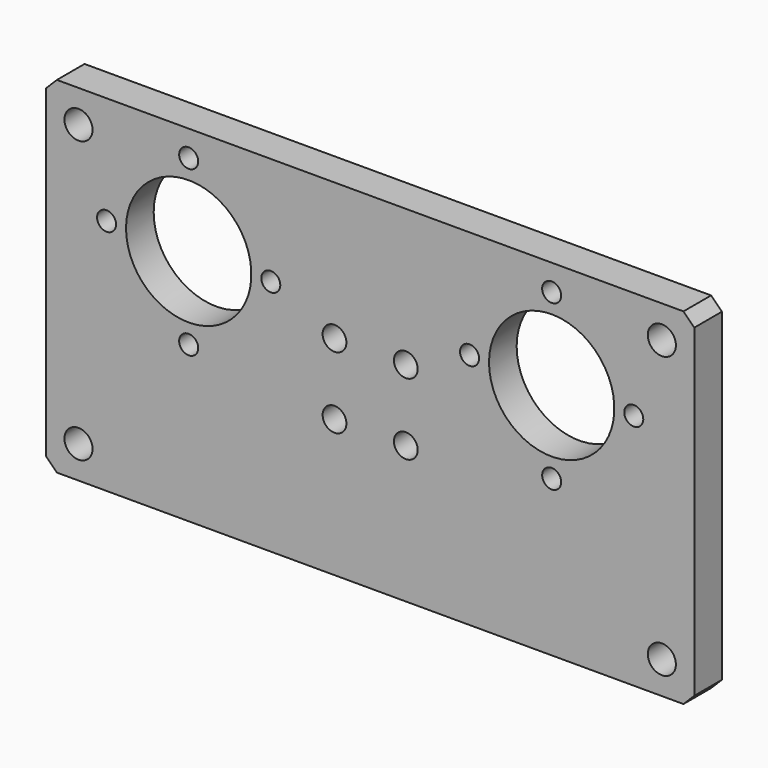
from build123d import *

# Parameters (mm, degrees)
F0_W             = 150
F0_H             = 80
F1_DEPTH         = 8
F2_SIZE          = 2.5
F4_D             = 4.4
F4_COPIES_COUNT  = 4
F4_COPIES2_COUNT = 2
F4_COPIES2_PITCH = 104.737768
F4_COPIES3_COUNT = 2
F4_COPIES3_PITCH = 92.195445
F4_COPIES4_COUNT = 2
F4_COPIES4_PITCH = 67.720012
F5_D             = 6.5
F6_D             = 5.5
F7_D             = 29


# Not quite as in the source:
# - a pattern or mirror of a feature is missing from the dataset's text; its kind, count and spacing are read off the source's solid


with BuildPart() as f1:
    # F0 (on Front) → F1 (new body)
    with BuildSketch(Plane.XZ):
        Rectangle(F0_W, F0_H)
    extrude(amount=F1_DEPTH)

    # F2
    f2_edges = [f1.edges().sort_by_distance(p)[0] for p in [
        (75, -4, 40),
        (75, -4, -40),
        (-75, -4, 40),
        (-75, -4, -40),
    ]]
    chamfer(f2_edges, length=F2_SIZE)

    # F4 (through all)
    with Locations(Plane.XZ.offset(8)):
        with Locations((42, 34)):
            f4 = Hole(F4_D / 2)

    # F4_copies: F4 ×4 about axis
    f4_copies_axis = Axis((42, 0, 15), (0, 1, 0))
    for i in range(1, F4_COPIES_COUNT):
        add(f4.rotate(f4_copies_axis, i * 360 / F4_COPIES_COUNT), mode=Mode.SUBTRACT)

    # F4_copies1: F4 across plane
    add(f4.mirror(Plane(origin=(0, 0, 0), x_dir=(0, 0, -1), z_dir=(-1, 0, 0))), mode=Mode.SUBTRACT)

    # F4_copies2: F4 ×2
    with Locations(*[Vector(-0.9834083939, 0, -0.1814054319) * (i * F4_COPIES2_PITCH) for i in range(1, F4_COPIES2_COUNT)]):
        add(f4, mode=Mode.SUBTRACT)

    # F4_copies3: F4 ×2
    with Locations(*[Vector(-0.9111079228, 0, -0.4121678699) * (i * F4_COPIES3_PITCH) for i in range(1, F4_COPIES3_COUNT)]):
        add(f4, mode=Mode.SUBTRACT)

    # F4_copies4: F4 ×2
    with Locations(*[Vector(-0.9598344457, 0, -0.2805669918) * (i * F4_COPIES4_PITCH) for i in range(1, F4_COPIES4_COUNT)]):
        add(f4, mode=Mode.SUBTRACT)

    # F5 (through all)
    with Locations(Plane.XZ.offset(8)):
        with Locations((67.5, 32.5), (67.5, -32.5), (-67.5, -32.5), (-67.5, 32.5)):
            Hole(F5_D / 2)

    # F6 (through all)
    with Locations(Plane.XZ.offset(8)):
        with Locations((-8.25, -8.25), (8.25, -8.25), (8.25, 8.25), (-8.25, 8.25)):
            Hole(F6_D / 2)

    # F7 (through all)
    with Locations(Plane.XZ.offset(8)):
        with Locations((-42, 15), (42, 15)):
            Hole(F7_D / 2)


solid = f1.part
